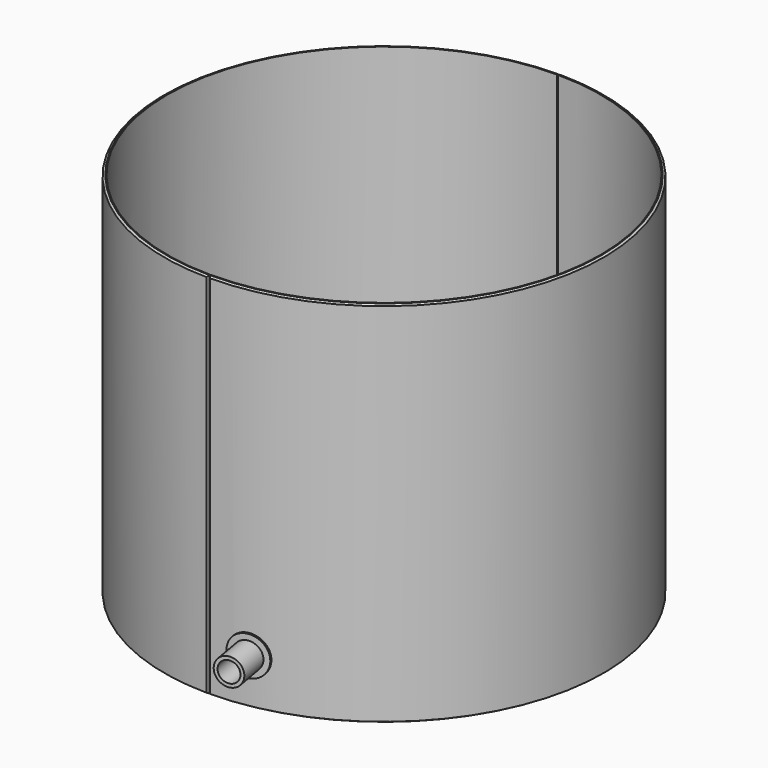
from build123d import *

# Parameters (mm, degrees)
F1_DEPTH  = 600
F5_DEPTH  = 600
F6_W      = 1537.0067954063
F6_H      = 1342.1749472618
F6_R      = 88.9
F7_DEPTH  = 1500
F8_R      = 70.65
F8_R_2    = 54.77
F9_DEPTH  = 1500
F10_DEPTH = 822
F13_DEPTH = 600
F12_W     = 975.8136421442
F12_H     = 1313.313126564
F12_R     = 63.5
F14_DEPTH = 800
F12_R_2   = 44.45
F12_R_3   = 33.32
F15_DEPTH = 900
F16_DEPTH = 800
F17_DEPTH = 822
F18_R     = 706
F19_DEPTH = 600


# Not quite as in the source:
# - a feature of the source that left no trace in its solid (it failed there, or was rolled back) is left out


with BuildPart() as f1:
    # F0 (on Top) → F1 (new body, symmetric)
    with BuildSketch(Plane.XY):
        with BuildLine():
            Line((-1.5, 708.9984132563), (-5.5300381047, 715.9786440101))
            ThreePointArc((-5.5300381047, 715.9786440101), (-716, 0), (-5.5300381047, -715.9786440101))
            Line((-5.5300381047, -715.9786440101), (-1.5, -708.9984132563))
            Line((-1.5, -708.9984132563), (-1.5, -705.9984065138))
            ThreePointArc((-1.5, -705.9984065138), (-706, 0), (-1.5, 705.9984065138))
            Line((-1.5, 705.9984065138), (-1.5, 708.9984132563))
        make_face()
    extrude(amount=F1_DEPTH, both=True)


with BuildPart() as f1b:
    # F0 (on Top) → F1, piece 2 (new body, symmetric)
    with BuildSketch(Plane.XY):
        with BuildLine():
            Line((5.5300381047, 715.9786440101), (1.5, 708.9984132563))
            Line((1.5, 708.9984132563), (1.5, 705.9984065138))
            ThreePointArc((1.5, 705.9984065138), (706, 0), (1.5, -705.9984065138))
            Line((1.5, -705.9984065138), (1.5, -708.9984132563))
            Line((1.5, -708.9984132563), (5.5300381047, -715.9786440101))
            ThreePointArc((5.5300381047, -715.9786440101), (716, 0), (5.5300381047, 715.9786440101))
        make_face()
    extrude(amount=F1_DEPTH, both=True)


with BuildPart() as f3_tool:
    # F2 (on Right) → F3 (revolve)
    with BuildSketch(Plane.YZ):
        Polygon((-726.7167568207, 589.7703095735), (-708.9984132563, 600), (-726.7167568207, 600), align=None)
        Polygon((-726.7167568207, -589.7703095735), (-726.7167568207, -600), (-708.9984132563, -600), align=None)
    revolve(axis=Axis((0, 0, -16.8183147907), (0, 0, -1)))


with BuildPart() as f1_1:
    add(f1.part)

    # F3: cut by f3_tool
    add(f3_tool.part, mode=Mode.SUBTRACT)

    # F2 (on Right) → F4 (revolve, cut)
    with BuildSketch(Plane.YZ):
        Polygon((-726.7167568207, 589.7703095735), (-708.9984132563, 600), (-726.7167568207, 600), align=None)
        Polygon((-726.7167568207, -589.7703095735), (-726.7167568207, -600), (-708.9984132563, -600), align=None)
    revolve(axis=Axis((0, 0, -16.8183147907), (0, 0, -1)), mode=Mode.SUBTRACT)


with BuildPart() as f1b_1:
    add(f1b.part)

    # F3: cut by f3_tool
    add(f3_tool.part, mode=Mode.SUBTRACT)


with BuildPart() as f5:
    # F0 (on Top) → F5 (new body, symmetric)
    with BuildSketch(Plane.XY):
        with BuildLine():
            ThreePointArc((-5.5300381047, -715.9786440101), (-716, 0), (-5.5300381047, 715.9786440101))
            Line((-5.5300381047, 715.9786440101), (-5.5763792061, 721.9784650493))
            ThreePointArc((-5.5763792061, 721.9784650493), (-722, 0), (-5.5763792061, -721.9784650493))
            Line((-5.5763792061, -721.9784650493), (-5.5300381047, -715.9786440101))
        make_face()
    extrude(amount=F5_DEPTH, both=True)

    # F6 (on Right) → F7 (cut)
    with BuildSketch(Plane.YZ):
        with Locations((-12.5137865543, 14.8827731609)):
            Rectangle(F6_W, F6_H)
        with Locations((0, -450)):
            Circle(F6_R, mode=Mode.SUBTRACT)
    extrude(amount=-F7_DEPTH, mode=Mode.SUBTRACT)


with BuildPart() as f9_tool:
    # F8 (on Right) → F9 (new body)
    with BuildSketch(Plane.YZ):
        with Locations((0, -450)):
            Circle(F8_R)
        with Locations((0, -450)):
            Circle(F8_R_2, mode=Mode.SUBTRACT)
        with Locations((0, -450)):
            Circle(F8_R_2)
    extrude(amount=-F9_DEPTH)


with BuildPart() as f1_2:
    add(f1_1.part)

    # F9: cut by f9_tool
    add(f9_tool.part, mode=Mode.SUBTRACT)

    # F12 (on line) → F16 (cut)
    with BuildSketch(Plane(origin=(0, 0, 0), x_dir=(-0.984807753, -0.1736481777, 0), z_dir=(-0.1736481777, 0.984807753, 0))):
        with Locations((0, -450)):
            Circle(F12_R_2)
        with Locations((0, -450)):
            Circle(F12_R_3, mode=Mode.SUBTRACT)
        with Locations((0, -450)):
            Circle(F12_R_3)
    extrude(amount=-F16_DEPTH, mode=Mode.SUBTRACT)


with BuildPart() as f5_1:
    add(f5.part)

    # F9: cut by f9_tool
    add(f9_tool.part, mode=Mode.SUBTRACT)


with BuildPart() as f10:
    # F8 (on Right) → F10 (new body)
    with BuildSketch(Plane.YZ):
        with Locations((0, -450)):
            Circle(F8_R)
        with Locations((0, -450)):
            Circle(F8_R_2, mode=Mode.SUBTRACT)
    extrude(amount=-F10_DEPTH)


with BuildPart() as f13:
    # F0 (on Top) → F13 (new body, symmetric)
    with BuildSketch(Plane.XY):
        with BuildLine():
            Line((5.5763792061, 721.9784650493), (5.5300381047, 715.9786440101))
            ThreePointArc((5.5300381047, 715.9786440101), (716, 0), (5.5300381047, -715.9786440101))
            Line((5.5300381047, -715.9786440101), (5.5763792061, -721.9784650493))
            ThreePointArc((5.5763792061, -721.9784650493), (722, 0), (5.5763792061, 721.9784650493))
        make_face()
    extrude(amount=F13_DEPTH, both=True)


with BuildPart() as f14_tool:
    # F12 (on line) → F14 (new body, symmetric)
    with BuildSketch(Plane(origin=(0, 0, 0), x_dir=(-0.984807753, -0.1736481777, 0), z_dir=(-0.1736481777, 0.984807753, 0))):
        with Locations((-264.7637650371, -22.878408432)):
            Rectangle(F12_W, F12_H)
        with Locations((0, -450)):
            Circle(F12_R, mode=Mode.SUBTRACT)
    extrude(amount=F14_DEPTH, both=True)


with BuildPart() as f10_1:
    add(f10.part)

    # F14: cut by f14_tool
    add(f14_tool.part, mode=Mode.SUBTRACT)


with BuildPart() as f13_1:
    add(f13.part)

    # F14: cut by f14_tool
    add(f14_tool.part, mode=Mode.SUBTRACT)


with BuildPart() as f15_tool:
    # F12 (on line) → F15 (new body)
    with BuildSketch(Plane(origin=(0, 0, 0), x_dir=(-0.984807753, -0.1736481777, 0), z_dir=(-0.1736481777, 0.984807753, 0))):
        with Locations((0, -450)):
            Circle(F12_R_2)
        with Locations((0, -450)):
            Circle(F12_R_3, mode=Mode.SUBTRACT)
        with Locations((0, -450)):
            Circle(F12_R_3)
    extrude(amount=-F15_DEPTH)


with BuildPart() as f1b_2:
    add(f1b_1.part)

    # F15: cut by f15_tool
    add(f15_tool.part, mode=Mode.SUBTRACT)


with BuildPart() as f10_2:
    add(f10_1.part)

    # F15: cut by f15_tool
    add(f15_tool.part, mode=Mode.SUBTRACT)


with BuildPart() as f13_2:
    add(f13_1.part)

    # F15: cut by f15_tool
    add(f15_tool.part, mode=Mode.SUBTRACT)


with BuildPart() as f17:
    # F12 (on line) → F17 (new body)
    with BuildSketch(Plane(origin=(0, 0, 0), x_dir=(-0.984807753, -0.1736481777, 0), z_dir=(-0.1736481777, 0.984807753, 0))):
        with Locations((0, -450)):
            Circle(F12_R_2)
        with Locations((0, -450)):
            Circle(F12_R_3, mode=Mode.SUBTRACT)
    extrude(amount=-F17_DEPTH)


with BuildPart() as f19_tool:
    # F18 (on Top) → F19 (new body)
    with BuildSketch(Plane.XY):
        Circle(F18_R)
    extrude(amount=-F19_DEPTH)


with BuildPart() as f10_3:
    add(f10_2.part)

    # F19: cut by f19_tool
    add(f19_tool.part, mode=Mode.SUBTRACT)


with BuildPart() as f17_1:
    add(f17.part)

    # F19: cut by f19_tool
    add(f19_tool.part, mode=Mode.SUBTRACT)


solid = Compound([f1_2.part, f5_1.part, f1b_2.part, f13_2.part, f10_3.part, f17_1.part])
